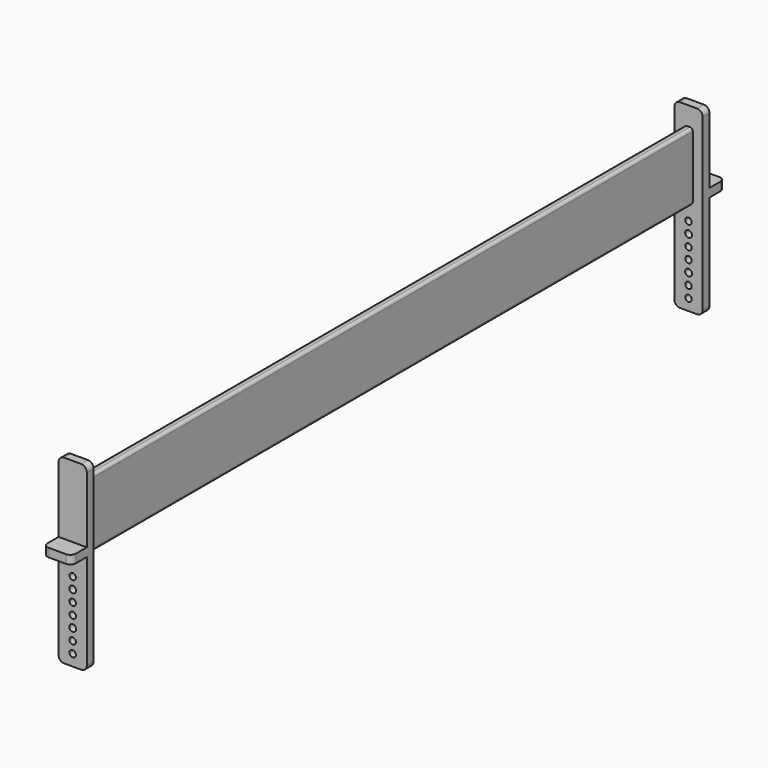
from build123d import *

# Parameters (mm, degrees)
F0_W     = 15.875
F0_H     = 101.6
F4_DEPTH = 4.7625
F2_W     = 15.875
F2_H     = 4.7625
F5_DEPTH = 10.795
F1_W     = 4.7625
F1_H     = 38.1
F6_DEPTH = 431.8
F7_START = 431.8
F7_DEPTH = 4.7625
F8_START = 436.5625
F8_DEPTH = 10.795
F3_R     = 1.905
F3_R_2   = 1.8018515142
F3_R_3   = 1.8092820601
F9_DEPTH = 447.3585
F11_R    = 1.5875
F12_R    = 3.175


with BuildPart() as f4:
    # F0 (on Front) → F4 (new body)
    with BuildSketch(Plane.XZ):
        Rectangle(F0_W, F0_H)
    extrude(amount=F4_DEPTH)

    # F2 (on Front) → F5 (join)
    with BuildSketch(Plane.XZ):
        with Locations((0, 8.28675)):
            Rectangle(F2_W, F2_H)
    extrude(amount=-F5_DEPTH)

    # F1 (on Front) → F6 (join)
    with BuildSketch(Plane.XZ):
        with Locations((0, 21.2725)):
            Rectangle(F1_W, F1_H)
    extrude(amount=F6_DEPTH)

    # F0 (on Front) → F7 (join)
    with BuildSketch(Plane.XZ.offset(F7_START)):
        Rectangle(F0_W, F0_H)
    extrude(amount=F7_DEPTH)

    # F2 (on Front) → F8 (join)
    with BuildSketch(Plane.XZ.offset(F8_START)):
        with Locations((0, 8.28675)):
            Rectangle(F2_W, F2_H)
    extrude(amount=F8_DEPTH)

    # F3 (on Front) → F9 (cut, through all)
    with BuildSketch(Plane.XZ):
        with Locations((0, -31.75)):
            Circle(F3_R)
        with Locations((0, -38.1)):
            Circle(F3_R_2)
        with Locations((0, -44.45)):
            Circle(F3_R_3)
        with Locations((0, -12.7)):
            Circle(F3_R)
        with Locations((0, -19.05)):
            Circle(F3_R_2)
        with Locations((0, -25.4)):
            Circle(F3_R_3)
        with Locations((0, -6.35)):
            Circle(F3_R_2)
    extrude(amount=F9_DEPTH, mode=Mode.SUBTRACT)

    # F11
    f11_edges = [f4.edges().sort_by_distance(p)[0] for p in [
        (-2.38125, -218.28125, 40.3225),
        (2.38125, -218.28125, 40.3225),
        (2.38125, -218.28125, 2.2225),
        (-2.38125, -218.28125, 2.2225),
    ]]
    fillet(f11_edges, radius=F11_R)

    # F12
    f12_edges = [f4.edges().sort_by_distance(p)[0] for p in [
        (7.9375, -434.18125, 50.8),
        (-7.9375, -434.18125, 50.8),
        (7.9375, -434.18125, -50.8),
        (-7.9375, -434.18125, -50.8),
        (-7.9375, -447.3575, 8.28675),
        (7.9375, -447.3575, 8.28675),
        (7.9375, -2.38125, 50.8),
        (-7.9375, -2.38125, 50.8),
        (7.9375, -2.38125, -50.8),
        (-7.9375, -2.38125, -50.8),
        (-7.9375, 10.795, 8.28675),
        (7.9375, 10.795, 8.28675),
    ]]
    fillet(f12_edges, radius=F12_R)


solid = f4.part
